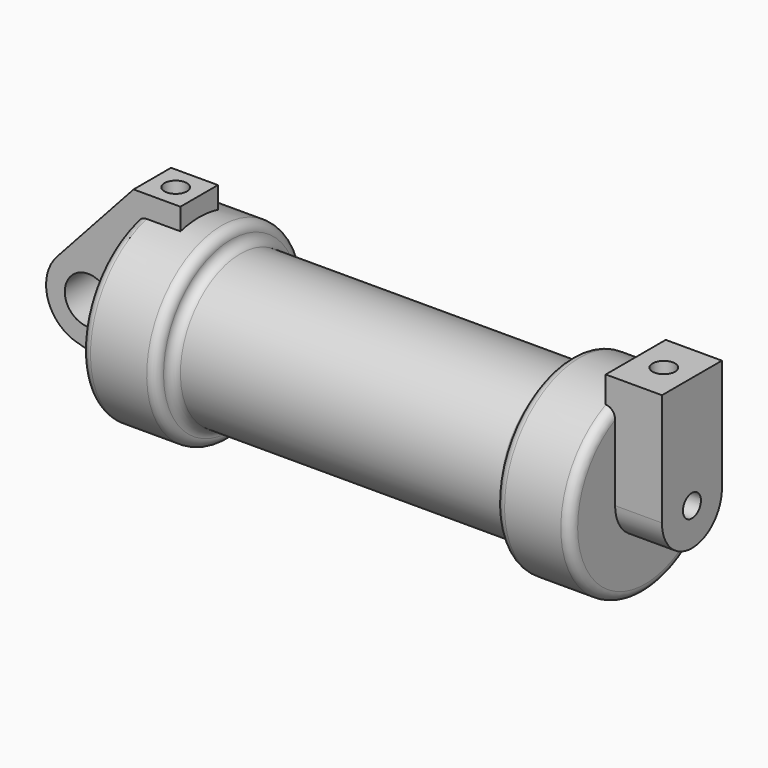
from build123d import *

# Parameters (mm, degrees)
F0_W          = 5.842
F0_H          = 12.7
F0_R          = 3.175
F2_DEPTH      = 3.175
F3_R          = 1.524
F4_DEPTH      = 6.35
F4_DEPTH_BACK = 1.27
F5_DEPTH      = 56.134
F6_R          = 1.524
F7_DEPTH      = 17.78
F8_DEPTH      = 10.414
F9_R          = 1.26999


# Not quite as in the source:
# - a fillet or chamfer is up to 0.001 mm smaller than in the source, because OpenCascade refuses the exact size


with BuildPart() as f1:
    # F0 (on Front) → F1 (revolve)
    with BuildSketch(Plane.XZ):
        with Locations((2.921, 6.35)):
            Rectangle(F0_W, F0_H)
        Polygon((5.842, 12.7), (5.842, 0), (66.294, 0), (66.294, 12.7), (56.134, 12.7), (56.134, 10.16), (10.16, 10.16), (10.16, 12.7), align=None)
    revolve(axis=Axis((33.147, 0, 0), (-1, 0, 0)))

    # F0 (on Front) → F2 (join, symmetric)
    with BuildSketch(Plane.XZ):
        with BuildLine():
            Line((-0.9398, 0), (0, 0))
            Line((0, 0), (0, 12.7))
            Line((0, 12.7), (5.842, 12.7))
            Line((5.842, 12.7), (5.842, 15.24))
            Line((5.842, 15.24), (-0.508, 15.24))
            Line((-0.508, 15.24), (-10.8806298187, 3.8475430269))
            ThreePointArc((-10.8806298187, 3.8475430269), (-4.5919612295, 5.3297205562), (-0.9398, 0))
        make_face()
        with Locations((2.921, 6.35)):
            Rectangle(F0_W, F0_H)
        with BuildLine():
            Line((5.842, 0), (0, 0))
            Line((0, 0), (-0.9398, 0))
            ThreePointArc((-0.9398, 0), (-3.1957909266, -4.5493385486), (-8.1826630726, -5.5069827884))
            Line((-8.1826630726, -5.5069827884), (5.842, -9.398))
            Line((5.842, -9.398), (5.842, 0))
        make_face()
        with BuildLine():
            ThreePointArc((-8.1826630726, -5.5069827884), (-3.1957909266, -4.5493385486), (-0.9398, 0))
            ThreePointArc((-0.9398, 0), (-4.5919612295, 5.3297205562), (-10.8806298187, 3.8475430269))
            ThreePointArc((-10.8806298187, 3.8475430269), (-12.1459778134, -1.5837270034), (-8.1826630726, -5.5069827884))
        make_face()
        with Locations((-6.6548, 0)):
            Circle(F0_R, mode=Mode.SUBTRACT)
    extrude(amount=F2_DEPTH, both=True)

    # F3 (on face) → F4 (join, two sides)
    with BuildSketch(Plane.YZ.offset(66.294)) as f4_sk:
        with BuildLine():
            ThreePointArc((-5.08, 0), (0, -5.08), (5.08, 0))
            ThreePointArc((5.08, 0), (0, 5.08), (-5.08, 0))
        make_face()
        Circle(F3_R, mode=Mode.SUBTRACT)
        with BuildLine():
            ThreePointArc((-5.08, 11.6397422652), (0, 12.7), (5.08, 11.6397422652))
            Line((5.08, 11.6397422652), (5.08, 15.24))
            Line((5.08, 15.24), (-5.08, 15.24))
            Line((-5.08, 15.24), (-5.08, 11.6397422652))
        make_face()
        with BuildLine():
            ThreePointArc((-5.08, 0), (0, 5.08), (5.08, 0))
            Line((5.08, 0), (5.08, 11.6397422652))
            ThreePointArc((5.08, 11.6397422652), (0, 12.7), (-5.08, 11.6397422652))
            Line((-5.08, 11.6397422652), (-5.08, 0))
        make_face()
    extrude(amount=F4_DEPTH)
    extrude(f4_sk.sketch, amount=-F4_DEPTH_BACK)

    # F5 (cut, through all): a face of the model
    f5_faces = [f1.faces().sort_by_distance(p)[0] for p in [
        (66.294, 0, 0),
    ]]
    extrude(f5_faces, amount=-F5_DEPTH, mode=Mode.SUBTRACT)

    # F6 (on face) → F7 (cut)
    with BuildSketch(Plane.XY.offset(15.24)):
        with Locations((2.667, 0)):
            Circle(F6_R)
    extrude(amount=-F7_DEPTH, mode=Mode.SUBTRACT)

    # F6 (on face) → F8 (cut)
    with BuildSketch(Plane.XY.offset(15.24)):
        with Locations((68.834, 0)):
            Circle(F6_R)
    extrude(amount=-F8_DEPTH, mode=Mode.SUBTRACT)

    # F9 (radius 1.27 in the source; OpenCascade refuses exactly that, so slightly less here)
    f9_edges = [f1.edges().sort_by_distance(p)[0] for p in [
        (10.16, 0, -12.7),
        (56.134, 0, -12.7),
        (10.16, 0, -10.16),
        (56.134, 0, -10.16),
        (66.294, 0, -12.7),
        (0, 0, -12.7),
    ]]
    fillet(f9_edges, radius=F9_R)


solid = f1.part
